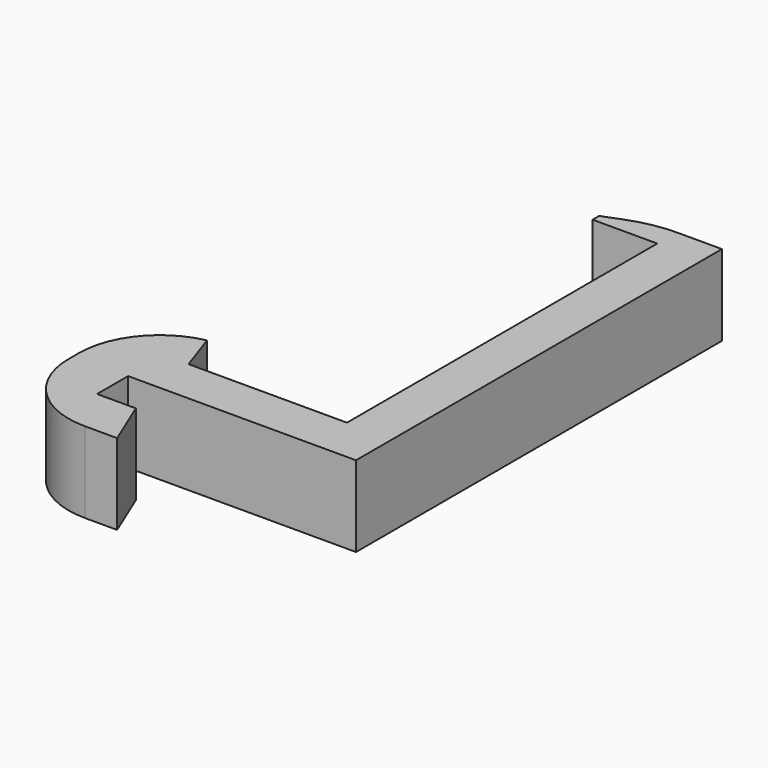
from build123d import *

# Parameters (mm, degrees)
F1_DEPTH    = 5
F2_T1_DEPTH = 29.4948974279
F2_T3_DEPTH = 30


# Not quite as in the source:
# - a fillet or chamfer that OpenCascade refuses, or shapes differently, is made with other operations: its cross-section is extruded or revolved along the edge and cut away or added


with BuildPart() as f1:
    # F0 (on Top) → F1 (new body)
    with BuildSketch(Plane.XY):
        with BuildLine():
            Line((-17.4608190332, -5.4), (-10.4608190332, -5.4))
            Line((-10.4608190332, -5.4), (-11.7008190332, -2.4))
            Line((-11.7008190332, -2.4), (-14.1008190332, -2.4))
            Line((-14.1008190332, -2.4), (-14.1008190332, 0))
            Line((-14.1008190332, 0), (0, 0))
            Line((0, 0), (0, 28.3))
            Line((0, 28.3), (-2.7189972619, 28.3))
            ThreePointArc((-2.7189972619, 28.3), (-4.184287104, 28.1646631001), (-5.6, 27.7632314196))
            Line((-5.6, 27.7632314196), (-6.8, 27.3))
            Line((-6.8, 27.3), (-6.8, 26.8))
            Line((-6.8, 26.8), (-2.8, 26.8))
            Line((-2.8, 26.8), (-2.8, 2.8))
            Line((-2.8, 2.8), (-12.6, 2.8))
            Line((-12.6, 2.8), (-13.4608190332, 5.3))
            Line((-13.4608190332, 5.3), (-17.4608190332, 5.3))
            Line((-17.4608190332, 5.3), (-17.4608190332, -5.4))
        make_face()
    extrude(amount=F1_DEPTH)

    # F2: fillet of radius 5 on 2 edges, made by hand

    # F2_s2 → F2_t1 (cut)
    with BuildSketch(Plane.XY.offset(-12.2474487139)):
        with BuildLine():
            ThreePointArc((-13.4608190332, 5.3), (-16.3338023794, 3.5632981746), (-17.4608190332, 0.4010205144))
            Line((-17.4608190332, 0.4010205144), (-17.4608190332, 5.3))
            Line((-17.4608190332, 5.3), (-13.4608190332, 5.3))
        make_face()
    extrude(amount=F2_T1_DEPTH, mode=Mode.SUBTRACT)

    # F2_s4 → F2_t3 (cut)
    with BuildSketch(Plane.XY.offset(-12.5)):
        with BuildLine():
            ThreePointArc((-17.4608190332, -0.4), (-15.9963529392, -3.9355339059), (-12.4608190332, -5.4))
            Line((-12.4608190332, -5.4), (-17.4608190332, -5.4))
            Line((-17.4608190332, -5.4), (-17.4608190332, -0.4))
        make_face()
    extrude(amount=F2_T3_DEPTH, mode=Mode.SUBTRACT)


solid = f1.part
